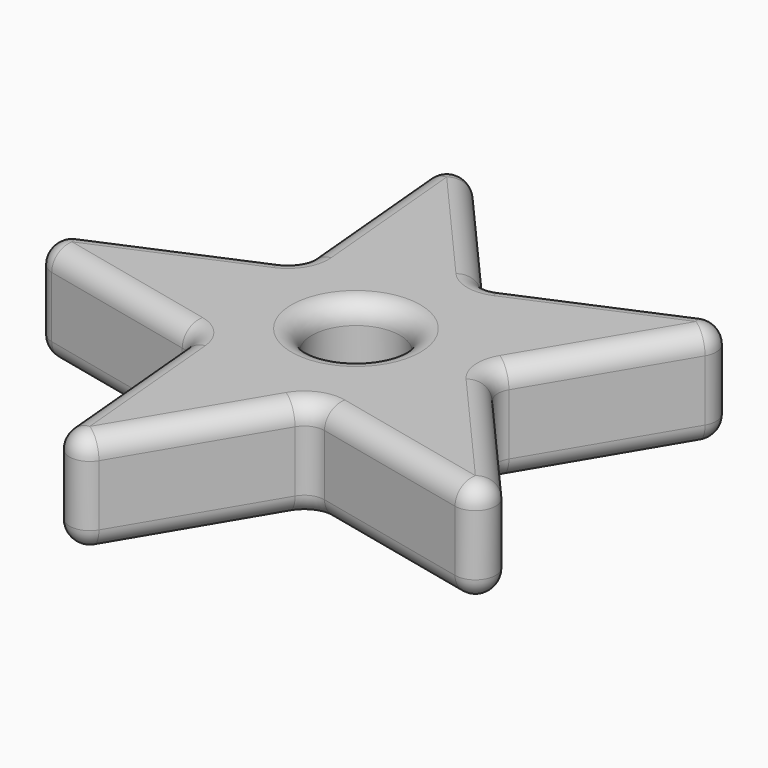
from build123d import *

# Parameters (mm, degrees)
F0_R     = 10.8505850545
F1_DEPTH = 12.5
F2_F1_R  = 5
F2_F2_R  = 5


with BuildPart() as f1:
    # F0 (on Top) → F1 (new body, symmetric)
    with BuildSketch(Plane.XY):
        Polygon((12.2831904488, -28.6552355439), (70.1120882045, -41.7908763236), (31.0484630838, 2.8270535563), align=None)
        Polygon((-18.079658483, -79.5946493517), (12.2831904488, -28.6552355439), (-23.4570338962, -20.5369630781), align=None)
        Polygon((-23.4570338962, -20.5369630781), (12.2831904488, -28.6552355439), (31.0484630838, 2.8270535563), (6.9058150355, 30.4024507297), (-26.7804346719, 15.962694336), align=None)
        Circle(F0_R, mode=Mode.SUBTRACT)
        Polygon((6.9058150355, 30.4024507297), (31.0484630838, 2.8270535563), (61.4113120156, 53.7664673641), align=None)
        Polygon((-81.2859316519, -7.4013222984), (-23.4570338962, -20.5369630781), (-26.7804346719, 15.962694336), align=None)
        Polygon((-26.7804346719, 15.962694336), (6.9058150355, 30.4024507297), (-32.1578100851, 75.0203806096), align=None)
    extrude(amount=F1_DEPTH, both=True)

    # F2: fillet of radius 5 on 22 edges, made by hand

    # F2_f1
    f2_f1_edges = [f1.edges().sort_by_distance(p)[0] for p in [
        (-23.4570338962, -20.5369630781, 0),
        (12.2831904488, -28.6552355439, 0),
        (31.0484630838, 2.8270535563, 0),
        (6.9058150355, 30.4024507297, 0),
        (-26.7804346719, 15.962694336, 0),
    ]]
    fillet(f2_f1_edges, radius=F2_F1_R)

    # F2_f2
    f2_f2_edges = [f1.edges().sort_by_distance(p)[0] for p in [
        (-81.2859316519, -7.4013222984, 0),
        (-18.079658483, -79.5946493517, 0),
        (70.1120882045, -41.7908763236, 0),
        (61.4113120156, 53.7664673641, 0),
        (-32.1578100851, 75.0203806096, 0),
        (-29.6338256066, 47.3004109145, 12.5),
        (-13.8224743676, 54.0780148962, 12.5),
        (47.1598689714, 29.8569799436, 12.5),
        (42.9688762969, -35.6253864896, 12.5),
        (-54.1427197444, -13.5668121324, 12.5),
        (-13.8224743676, 54.0780148962, -12.5),
        (-29.6338256066, 47.3004109145, -12.5),
        (-54.1427197444, -13.5668121324, -12.5),
        (-3.8282154389, -55.6851619313, -12.5),
        (51.7767524869, -20.8485106102, -12.5),
        (-10.8505850545, 0, 12.5),
        (-10.8505850545, 0, -12.5),
        (32.2239403022, 2.9340842019, -12.5),
        (12.7482250787, -29.7401065238, -12.5),
        (-24.3451039073, -21.3144808627, -12.5),
        (-27.7943267531, 16.5670328981, -12.5),
        (7.1672652795, 31.5534702865, -12.5),
        (-24.3451039073, -21.3144808627, 12.5),
        (12.7482250787, -29.7401065238, 12.5),
        (32.2239403022, 2.9340842019, 12.5),
        (7.1672652795, 31.5534702865, 12.5),
        (-27.7943267531, 16.5670328981, 12.5),
    ]]
    fillet(f2_f2_edges, radius=F2_F2_R)


solid = f1.part
